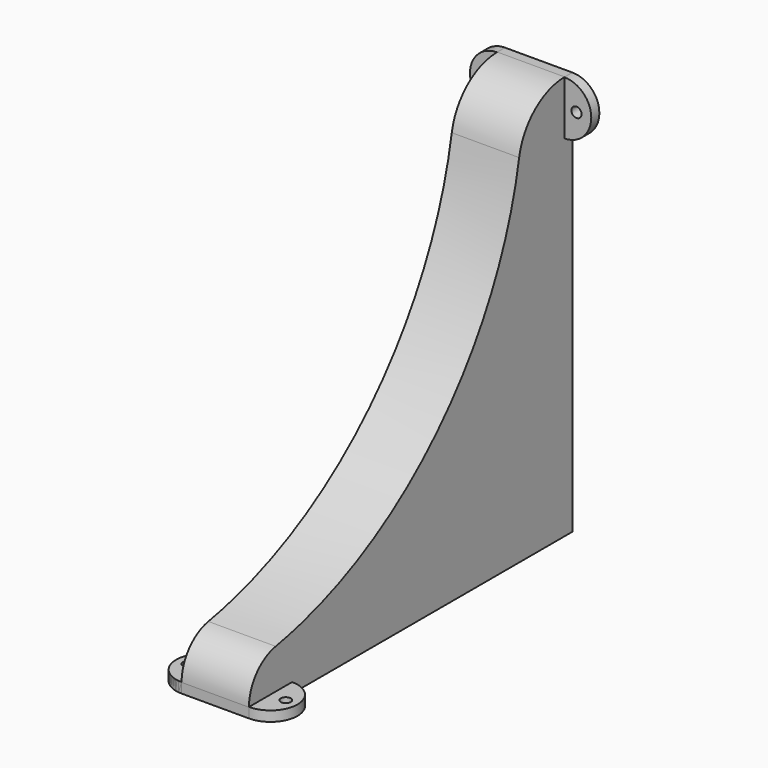
from build123d import *

# Parameters (mm, degrees)
F1_DEPTH     = 15
F0_R         = 1.5
F2_DEPTH     = 3
F0_W         = 2
F0_H         = 3
F3_DEPTH     = 120
F4_DEPTH     = 120
F5_W         = 3
F5_H         = 16
F6_DEPTH     = 17
F8_DEPTH     = 3
F7_R         = 1.5
F9_DEPTH     = 3
F12_T1_DEPTH = 105.7045814642
F13_T1_DEPTH = 80.3553390593
F14_R        = 112.0195092941


# Not quite as in the source:
# - a fillet or chamfer that OpenCascade refuses, or shapes differently, is made with other operations: its cross-section is extruded or revolved along the edge and cut away or added
# - a feature names something its author has since deleted; it is built from what else it names


with BuildPart() as f1:
    # F0 (on Top) → F1 (new body)
    with BuildSketch(Plane.XY):
        Polygon((-8, 44.9565169007), (-10, 44.9565169007), (-10, -39.0434830993), (-10, -55.0434830993), (-8, -55.0434830993), align=None)
        Polygon((10, -39.0434830993), (10, 44.9565169007), (-8, 44.9565169007), (-8, -55.0434830993), (10, -55.0434830993), align=None)
    extrude(amount=F1_DEPTH)

    # F0 (on Top) → F2 (join)
    with BuildSketch(Plane.XY):
        Polygon((10, -39.0434830993), (10, 44.9565169007), (-8, 44.9565169007), (-8, -55.0434830993), (10, -55.0434830993), align=None)
        with BuildLine():
            ThreePointArc((10, -55.0434830993), (18, -47.0434830993), (10, -39.0434830993))
            Line((10, -39.0434830993), (10, -55.0434830993))
        make_face()
        with Locations((14.5272817463, -47.0434830993)):
            Circle(F0_R, mode=Mode.SUBTRACT)
    extrude(amount=F2_DEPTH)

    # F0 (on Top) → F3 (join)
    with BuildSketch(Plane.XY):
        Polygon((10, 64.9565169007), (-8, 64.9565169007), (-8, 61.9565169007), (-8, 44.9565169007), (10, 44.9565169007), align=None)
        with Locations((-9, 63.4565169007)):
            Rectangle(F0_W, F0_H)
    extrude(amount=F3_DEPTH)

    # F0 (on Top) → F4 (join, through all)
    with BuildSketch(Plane.XY):
        with Locations((-9, 63.4565169007)):
            Rectangle(F0_W, F0_H)
    extrude(amount=F4_DEPTH)

    # F5 (on face) → F6 (join)
    with BuildSketch(Plane.YZ.offset(10)):
        with Locations((63.4565169007, 112)):
            Rectangle(F5_W, F5_H)
    extrude(amount=F6_DEPTH)

    # F7 (on face) → F8 (cut, through all)
    with BuildSketch(Plane.XZ.offset(-61.9565169007)):
        with BuildLine():
            ThreePointArc((10, 120), (18, 112), (10, 104))
            Line((10, 104), (27, 104))
            Line((27, 104), (27, 120))
            Line((27, 120), (10, 120))
        make_face()
    extrude(amount=-F8_DEPTH, mode=Mode.SUBTRACT)

    # F7 (on face) → F9 (cut, through all)
    with BuildSketch(Plane.XZ.offset(-61.9565169007)):
        with Locations((13.6100761592, 112)):
            Circle(F7_R)
    extrude(amount=-F9_DEPTH, mode=Mode.SUBTRACT)

    # F11: F1 across plane


with BuildPart() as f2:
    # F0 (on Top) → F2, piece 2 (new body)
    with BuildSketch(Plane.XY):
        with BuildLine():
            Line((-10, -55.0434830993), (-10, -39.0434830993))
            ThreePointArc((-10, -39.0434830993), (-18, -47.0434830993), (-10, -55.0434830993))
        make_face()
        with Locations((-14.5272817463, -47.0434830993)):
            Circle(F0_R, mode=Mode.SUBTRACT)
    extrude(amount=F2_DEPTH)


with BuildPart() as f1_1:
    add(f1.part)
    add(f1.part.mirror(Plane(origin=(0, 64.9565169007, 120), x_dir=(0, 1, 0), z_dir=(1, 0, 0))))

    # F12: fillet of radius 17.1409162928 on 1 edges, made by hand

    # F12_s2 → F12_t1 (cut)
    with BuildSketch(Plane.YZ.offset(-52.8522907321)):
        with BuildLine():
            ThreePointArc((44.9565169007, 102.8590837072), (49.9769750471, 114.9795418536), (62.0974331935, 120))
            Line((62.0974331935, 120), (44.9565169007, 120))
            Line((44.9565169007, 120), (44.9565169007, 102.8590837072))
        make_face()
    extrude(amount=F12_T1_DEPTH, mode=Mode.SUBTRACT)

    # F13: fillet of radius 12.0710678119 on 1 edges, made by hand

    # F13_s2 → F13_t1 (cut)
    with BuildSketch(Plane.YZ.offset(-40.1776695297)):
        with BuildLine():
            ThreePointArc((-55.0434830993, 2.9289321881), (-51.5079491934, 11.4644660941), (-42.9724152874, 15))
            Line((-42.9724152874, 15), (-55.0434830993, 15))
            Line((-55.0434830993, 15), (-55.0434830993, 2.9289321881))
        make_face()
    extrude(amount=F13_T1_DEPTH, mode=Mode.SUBTRACT)

    # F14
    f14_edges = [f1_1.edges().sort_by_distance(p)[0] for p in [
        (0, 44.956517, 15),
    ]]
    fillet(f14_edges, radius=F14_R)


solid = Compound([f2.part, f1_1.part])
